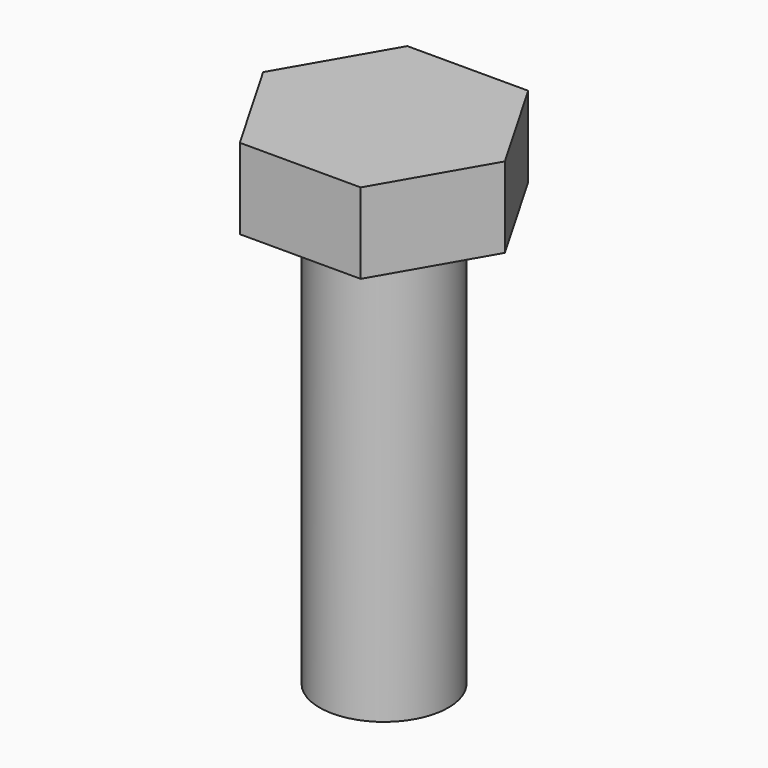
from build123d import *

# Parameters (mm, degrees)
F0_R     = 12.7
F1_DEPTH = 82.55
F3_DEPTH = 15.875


# Not quite as in the source:
# - a feature names something its author has since deleted; it is built from what else it names


with BuildPart() as f1:
    # F0 (on Top) → F1 (new body)
    with BuildSketch(Plane.XY):
        Circle(F0_R)
    extrude(amount=-F1_DEPTH)

    # F2 (on face) → F3 (join)
    with BuildSketch(Plane.XY):
        Polygon((11.9150661804, 20.6375), (-11.9150661804, 20.6375), (-23.8301323608, 0), (-11.9150661804, -20.6375), (11.9150661804, -20.6375), (23.8301323608, 0), align=None)
    extrude(amount=F3_DEPTH)


solid = f1.part
